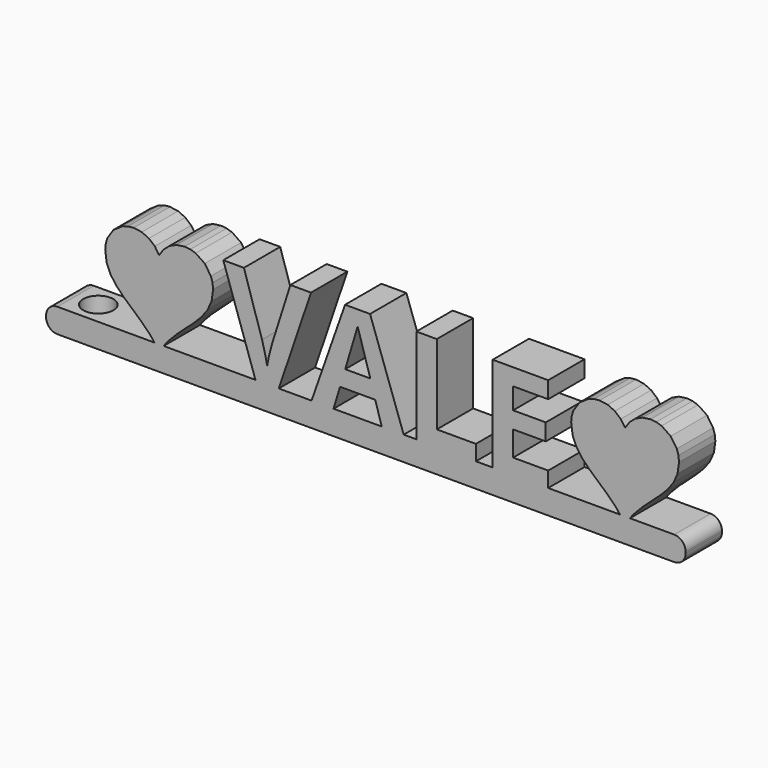
from build123d import *

# Parameters (mm, degrees)
F0_TEXT_SIZE = 17.8452958992
F1_DEPTH     = 3
F2_W         = 77
F2_H         = 6
F3_DEPTH     = 0.2
F4_DEPTH     = 3
F5_W         = 6
F5_H         = 3.2
F6_DEPTH     = 7.5
F7_R         = 1.5
F8_R         = 2
F9_DEPTH     = 4
F10_R        = 1.5


# Not quite as in the source:
# - Text() gives the source's letters only with a copy of the font that has no kerning and outlines rounded to 1/6400 em; it was checked with that copy


with BuildPart() as f1:
    # F0 (on Front) → F1 (new body, symmetric)
    with BuildSketch(Plane.XZ):
        Polygon((46.3078560556, 12.4433699982), (45.2468360556, 12.5970599982), (44.4882260556, 12.5204799982), (43.7814260556, 12.3008699982), (42.5840860556, 11.4933499982), (41.7764660556, 10.2961199982), (41.5568160556, 9.5893599982), (41.4802260556, 8.8307599982), (41.6687460556, 7.3860999982), (42.1894860556, 6.1597099982), (42.9752360556, 5.0814099982), (43.9587660556, 4.0810299982), (46.2556160556, 2.0250499982), (47.4402060556, 0.8247399982), (48.5631960556, -0.5860800018), (48.6074760556, -0.6500000018), (48.6505060556, -0.5851400018), (49.7284160556, 0.8234499982), (50.8917160556, 2.0333299982), (53.1953860556, 4.1212499982), (54.1961760556, 5.1327499982), (55.0011760556, 6.2116199982), (55.5375660556, 7.4226699982), (55.7325460556, 8.8307599982), (55.6559660556, 9.5893599982), (55.4363560556, 10.2961199982), (54.6288360556, 11.4933499982), (53.4316060556, 12.3008699982), (52.7248360556, 12.5204799982), (51.9662460556, 12.5970599982), (50.9052260556, 12.4433699982), (49.9641560556, 12.0123599982), (49.1842060556, 11.3491699982), (48.6065360556, 10.4989199982), (48.0288760556, 11.3491699982), (47.2489260556, 12.0123599982), align=None)
        Polygon((-15.2581707838, 12.5082299799), (-16.3191907838, 12.6619199799), (-17.0778007838, 12.5853399799), (-17.7846007838, 12.3657299799), (-18.9819407838, 11.5582099799), (-19.7895607838, 10.3609799799), (-20.0092107838, 9.6542199799), (-20.0858007838, 8.8956199799), (-19.8972807838, 7.4509599799), (-19.3765407838, 6.2245699799), (-18.5907907838, 5.1462699799), (-17.6072607838, 4.1458899799), (-15.3104107838, 2.0899099799), (-14.1258207838, 0.8895999799), (-13.0028307838, -0.5212200201), (-12.9585507838, -0.5851400201), (-12.9155207838, -0.5202800201), (-11.8376107838, 0.8883099799), (-10.6743107838, 2.0981899799), (-8.3706407838, 4.1861099799), (-7.3698507838, 5.1976099799), (-6.5648507838, 6.2764799799), (-6.0284607838, 7.4875299799), (-5.8334807838, 8.8956199799), (-5.9100607838, 9.6542199799), (-6.1296707838, 10.3609799799), (-6.9371907838, 11.5582099799), (-8.1344207838, 12.3657299799), (-8.8411907838, 12.5853399799), (-9.5997807838, 12.6619199799), (-10.6608007838, 12.5082299799), (-11.6018707838, 12.0772199799), (-12.3818207838, 11.4140299799), (-12.9594907838, 10.5637799799), (-13.5371507838, 11.4140299799), (-14.3171007838, 12.0772199799), align=None)
        with Locations((-4.489034181, 0)):
            Text('VALE', F0_TEXT_SIZE, font='Open Sans', font_style=FontStyle.BOLD, text_align=(TextAlign.LEFT, TextAlign.BOTTOM))
    extrude(amount=F1_DEPTH, both=True)



with BuildPart() as f3:
    # F2 (on Top) → F3 (new body)
    with BuildSketch(Plane.XY):
        with Locations((18.1, 0)):
            Rectangle(F2_W, F2_H)
    extrude(amount=F3_DEPTH)


with BuildPart() as f4:
    # F4 (new): a face of the model
    f4_faces = [f3.part.faces().sort_by_distance(p)[0] for p in [
        (18.1, 0, 0),
    ]]
    extrude(f4_faces, amount=F4_DEPTH)


with BuildPart() as f1_1:
    add(f1.part)

    add(f3.part)  # F6 merges F3

    add(f4.part)  # F6 merges F4
    # F5 (on face) → F6 (join)
    with BuildSketch(Plane(origin=(-20.4, 0, 0), x_dir=(0, -1, 0), z_dir=(-1, 0, 0))):
        with Locations((0, -1.4)):
            Rectangle(F5_W, F5_H)
    extrude(amount=F6_DEPTH)

    # F7
    f7_edges = [f1_1.edges().sort_by_distance(p)[0] for p in [
        (-27.9, 0, -3),
        (-27.9, 0, 0.2),
        (56.6, 0, -3),
    ]]
    fillet(f7_edges, radius=F7_R)

    # F8 (on face) → F9 (cut)
    with BuildSketch(Plane.XY.offset(0.2)):
        with Locations((-23.4, 0)):
            Circle(F8_R)
    extrude(amount=-F9_DEPTH, mode=Mode.SUBTRACT)

    # F10
    f10_edges = [f1_1.edges().sort_by_distance(p)[0] for p in [
        (56.6, 0, 0.2),
    ]]
    fillet(f10_edges, radius=F10_R)


solid = f1_1.part
